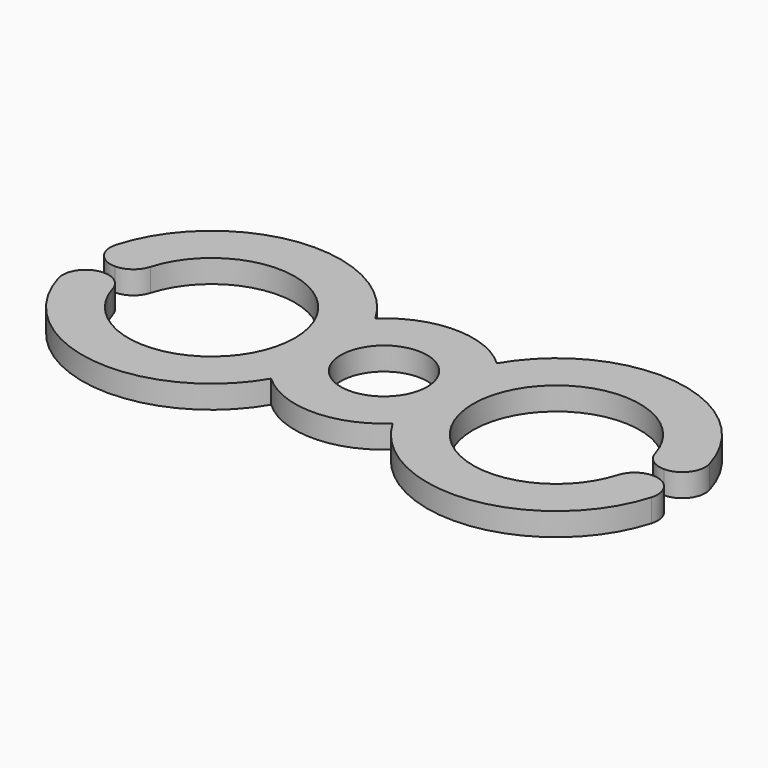
from build123d import *

# Parameters (mm, degrees)
F1_DEPTH = 1.27
F2_R     = 9.2075
F2_R_2   = 4.7625
F3_DEPTH = 25.4
F4_W     = 16.7551115155
F4_H     = 1.524
F5_DEPTH = 25.4
F6_R     = 2.53999


# Not quite as in the source:
# - a fillet or chamfer is up to 0.001 mm smaller than in the source, because OpenCascade refuses the exact size


with BuildPart() as f1:
    # F0 (on Top) → F1 (new body, symmetric)
    with BuildSketch(Plane.XY):
        with BuildLine():
            ThreePointArc((-6.7098333333, -7.2008987556), (-5.2579227906, -3.7297804895), (-4.7625, 0))
            ThreePointArc((-4.7625, 0), (-5.2579227906, 3.7297804895), (-6.7098333333, 7.2008987556))
            ThreePointArc((-6.7098333333, 7.2008987556), (-9.8425, 0), (-6.7098333333, -7.2008987556))
        make_face()
        with BuildLine():
            ThreePointArc((-6.7098333333, 7.2008987556), (-5.2579227906, 3.7297804895), (-4.7625, 0))
            ThreePointArc((-4.7625, 0), (-5.2579227906, -3.7297804895), (-6.7098333333, -7.2008987556))
            ThreePointArc((-6.7098333333, -7.2008987556), (0, -9.8425), (6.7098333333, -7.2008987556))
            ThreePointArc((6.7098333333, -7.2008987556), (4.7625, 0), (6.7098333333, 7.2008987556))
            ThreePointArc((6.7098333333, 7.2008987556), (0, 9.8425), (-6.7098333333, 7.2008987556))
        make_face()
        with BuildLine():
            ThreePointArc((-6.7098333333, -7.2008987556), (-9.8425, 0), (-6.7098333333, 7.2008987556))
            ThreePointArc((-6.7098333333, 7.2008987556), (-33.3375, 0), (-6.7098333333, -7.2008987556))
        make_face()
        with BuildLine():
            ThreePointArc((9.8425, 0), (9.0254180189, 3.9264024034), (6.7098333333, 7.2008987556))
            ThreePointArc((6.7098333333, 7.2008987556), (4.7625, 0), (6.7098333333, -7.2008987556))
            ThreePointArc((6.7098333333, -7.2008987556), (9.0254180189, -3.9264024034), (9.8425, 0))
        make_face()
        with BuildLine():
            ThreePointArc((33.3375, 0), (22.7797804895, 13.7920772094), (6.7098333333, 7.2008987556))
            ThreePointArc((6.7098333333, 7.2008987556), (9.0254180189, 3.9264024034), (9.8425, 0))
            ThreePointArc((9.8425, 0), (9.0254180189, -3.9264024034), (6.7098333333, -7.2008987556))
            ThreePointArc((6.7098333333, -7.2008987556), (22.7797804895, -13.7920772094), (33.3375, 0))
        make_face()
    extrude(amount=F1_DEPTH, both=True)

    # F2 (on face) → F3 (cut)
    with BuildSketch(Plane.XY.offset(1.27)):
        with Locations((-19.05, 0)):
            Circle(F2_R)
        with Locations((19.05, 0)):
            Circle(F2_R)
        Circle(F2_R_2)
    extrude(amount=-F3_DEPTH, mode=Mode.SUBTRACT)

    # F4 (on face) → F5 (cut)
    with BuildSketch(Plane.XY.offset(1.27)):
        with Locations((-24.9599442422, 0)):
            Rectangle(F4_W, F4_H)
        with Locations((24.9599442422, 0)):
            Rectangle(F4_W, F4_H)
    extrude(amount=-F5_DEPTH, mode=Mode.SUBTRACT)

    # F6 (radius 2.54 in the source; OpenCascade refuses exactly that, so slightly less here)
    f6_edges = [f1.edges().sort_by_distance(p)[0] for p in [
        (-33.317166, 0.762, 0),
        (-28.225915, 0.762, 0),
        (-28.225915, -0.762, 0),
        (-33.317166, -0.762, 0),
        (28.225915, -0.762, 0),
        (28.225915, 0.762, 0),
        (33.317166, 0.762, 0),
        (33.317166, -0.762, 0),
    ]]
    fillet(f6_edges, radius=F6_R)


solid = f1.part
